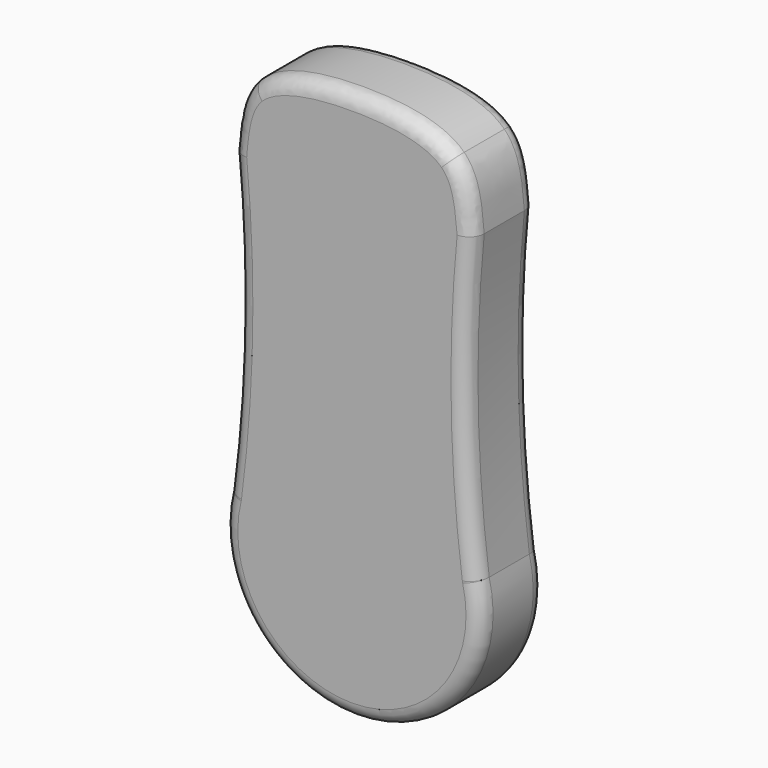
from build123d import *

# Parameters (mm, degrees)
F1_DEPTH = 16
F2_R     = 3
F3_R     = 3


with BuildPart() as f1:
    # F0 (on Front) → F1 (new body)
    with BuildSketch(Plane.XZ):
        with BuildLine():
            ThreePointArc((1, 92), (2.2082244019, 61.9715295933), (0, 32))
            ThreePointArc((0, 32), (25, 0), (50, 32))
            ThreePointArc((50, 32), (47.7917755981, 61.9715295933), (49, 92))
            Line((49, 92), (25, 92))
            Line((25, 92), (1, 92))
        make_face()
        with BuildLine():
            add(Edge.make_bspline(
                [(1, 92), (1.4186086824, 96.9319457504), (1.8372173648, 101.8638915008), (5, 105)],
                knots=[0, 0, 0, 0, 0.2241015784, 0.2241015784, 0.2241015784, 0.2241015784], degree=3))
            Line((1, 92), (25, 92))
            Line((25, 92), (25, 105))
            Line((25, 105), (5, 105))
        make_face()
        with BuildLine():
            Line((25, 92), (49, 92))
            add(Edge.make_bspline(
                [(45, 105), (48.1627826352, 101.8638915008), (48.5813913176, 96.9319457504), (49, 92)],
                knots=[0.7758984216, 0.7758984216, 0.7758984216, 0.7758984216, 1, 1, 1, 1], degree=3))
            Line((45, 105), (25, 105))
            Line((25, 105), (25, 92))
        make_face()
        with BuildLine():
            add(Edge.make_bspline(
                [(5, 105), (8.8938000478, 108.8609606896), (16.9469000239, 110), (25, 110)],
                knots=[0.2241015784, 0.2241015784, 0.2241015784, 0.2241015784, 0.5, 0.5, 0.5, 0.5], degree=3))
            Line((5, 105), (25, 105))
            Line((25, 105), (25, 110))
        make_face()
        with BuildLine():
            Line((25, 105), (45, 105))
            add(Edge.make_bspline(
                [(25, 110), (33.0530999761, 110), (41.1061999522, 108.8609606896), (45, 105)],
                knots=[0.5, 0.5, 0.5, 0.5, 0.7758984216, 0.7758984216, 0.7758984216, 0.7758984216], degree=3))
            Line((25, 110), (25, 105))
        make_face()
    extrude(amount=F1_DEPTH)

    # F2
    f2_edges = [f1.edges().sort_by_distance(p)[0] for p in [
        (2.208224, -16, 61.97153),
        (25, -16, 0),
        (47.791776, -16, 61.97153),
        (25, -16, 110),
    ]]
    fillet(f2_edges, radius=F2_R)

    # F3
    f3_edges = [f1.edges().sort_by_distance(p)[0] for p in [
        (2.208224, 0, 61.97153),
        (25, 0, 0),
        (47.791776, 0, 61.97153),
        (25, 0, 110),
    ]]
    fillet(f3_edges, radius=F3_R)


solid = f1.part
